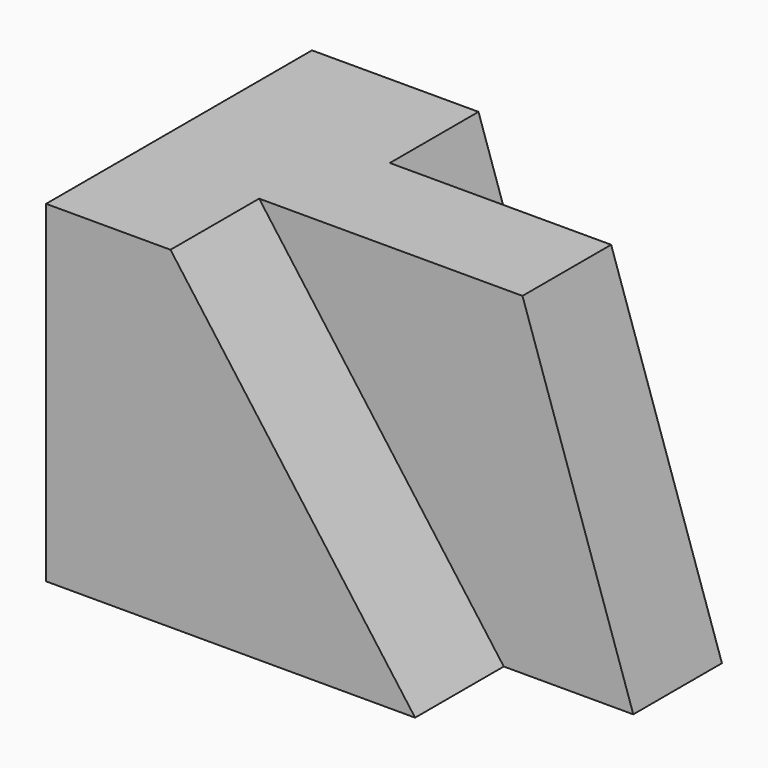
from build123d import *

# Parameters (mm, degrees)
F0_W     = 57.15
F0_H     = 38.1
F1_DEPTH = 38.1
F3_DEPTH = 38.1
F5_DEPTH = 12.7
F9_DEPTH = 12.7


# Not quite as in the source:
# - a feature of the source that left no trace in its solid (it failed there, or was rolled back) is left out
# - a feature names something its author has since deleted; it is built from what else it names


with BuildPart() as f1:
    # F0 (on Front) → F1 (new body)
    with BuildSketch(Plane.XZ):
        with Locations((28.575, 19.05)):
            Rectangle(F0_W, F0_H)
    extrude(amount=F1_DEPTH)

    # F2 (on face) → F3 (cut)
    with BuildSketch(Plane.XZ.offset(38.1)):
        Polygon((57.15, 38.1), (44.45, 38.1), (57.15, 0), align=None)
    extrude(amount=-F3_DEPTH, mode=Mode.SUBTRACT)

    # F4 (on Front) → F5 (cut)
    with BuildSketch(Plane.XZ):
        Polygon((44.4645239406, 38.2572661593), (19.05, 38.2047749953), (31.75, 0), (57.1819730103, 0), align=None)
    extrude(amount=F5_DEPTH, mode=Mode.SUBTRACT)

    # F7 (on face) → F9 (cut)
    with BuildSketch(Plane.XZ.offset(38.1)):
        Polygon((44.45, 38.1), (14.2616005614, 38.1), (42.3013567924, 0), (57.15, 0), align=None)
    extrude(amount=-F9_DEPTH, mode=Mode.SUBTRACT)


solid = f1.part
